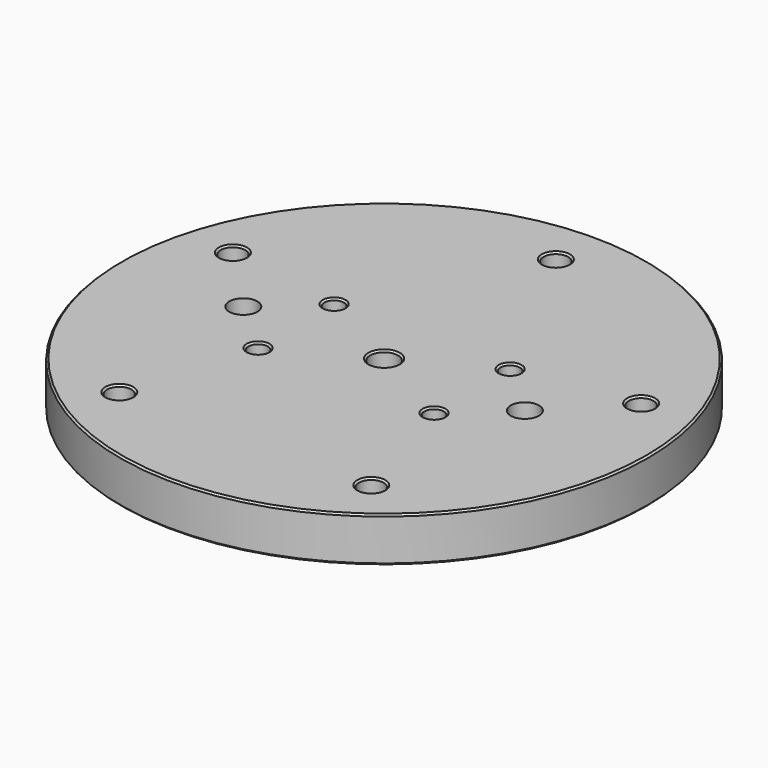
from build123d import *

# Parameters (mm, degrees)
F0_R           = 75
F1_DEPTH       = 12.7
F2_D           = 5.5
F2_CBORE_D     = 9.75
F2_CBORE_DEPTH = 5
F4_D           = 7
F5_D           = 7.9375
F6_SIZE        = 0.5
F8_D           = 8


# Not quite as in the source:
# - a length typed as a fraction of an inch, garbled in the dataset ("3 / 203.2 mm" for 3/8 in), is restored


with BuildPart() as f1:
    # F0 (on Top) → F1 (new body)
    with BuildSketch(Plane.XY):
        Circle(F0_R)
    extrude(amount=F1_DEPTH)

    # F2 (through all)
    with Locations(Plane(origin=(0, 0, 0), x_dir=(1, 0, 0), z_dir=(0, 0, -1))):
        with Locations((-25, 13.5), (25, 13.5), (-25, -13.5), (25, -13.5)):
            CounterBoreHole(F2_D / 2, F2_CBORE_D / 2, F2_CBORE_DEPTH)

    # F4 (through all)
    with Locations(Plane.XY.offset(12.7)):
        with Locations((0, 61), (58, 18.8), (-58, 18.8), (-35.8, -49.3), (35.8, -49.3)):
            Hole(F4_D / 2)

    # F5 (through all)
    with Locations(Plane(origin=(0, 0, 0), x_dir=(1, 0, 0), z_dir=(0, 0, -1))):
        with Locations((0, 0)):
            Hole(F5_D / 2)

    # F6
    f6_edges = [f1.edges().sort_by_distance(p)[0] for p in [
        (-75, 0, 0),
        (-39.3, -49.3, 0),
        (-29.875, -13.5, 0),
        (32.3, -49.3, 0),
        (20.125, -13.5, 0),
        (-3.96875, 0, 0),
        (-61.5, 18.8, 0),
        (-29.875, 13.5, 0),
        (20.125, 13.5, 0),
        (54.5, 18.8, 0),
        (-3.5, 61, 0),
        (-75, 0, 12.7),
        (-39.3, -49.3, 12.7),
        (-27.75, -13.5, 12.7),
        (32.3, -49.3, 12.7),
        (22.25, -13.5, 12.7),
        (-3.96875, 0, 12.7),
        (-61.5, 18.8, 12.7),
        (-27.75, 13.5, 12.7),
        (22.25, 13.5, 12.7),
        (54.5, 18.8, 12.7),
        (-3.5, 61, 12.7),
    ]]
    chamfer(f6_edges, length=F6_SIZE)

    # F8 (through all)
    with Locations(Plane.XY.offset(12.7)):
        with Locations((-40, 0), (40, 0)):
            Hole(F8_D / 2)


solid = f1.part
